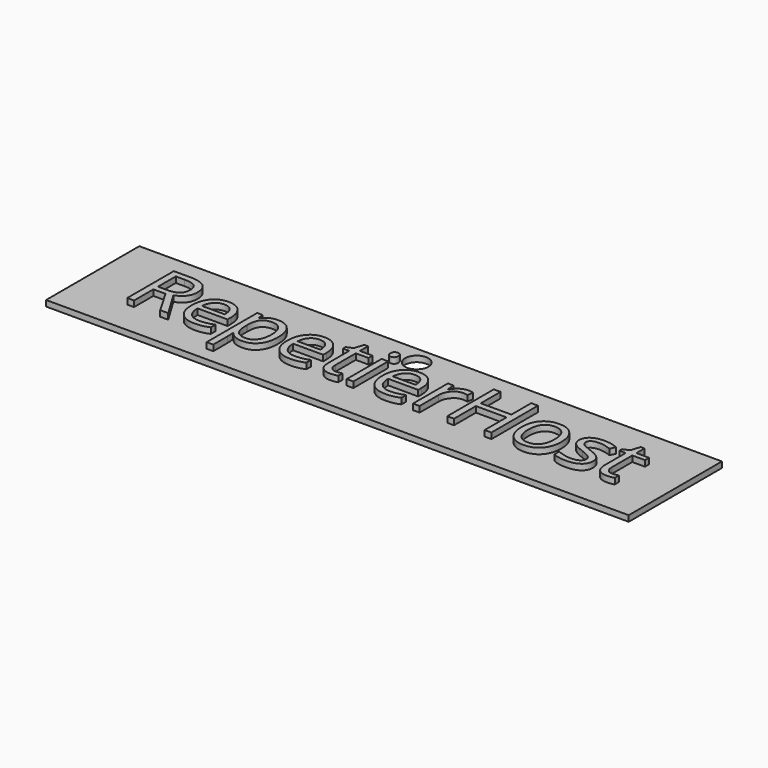
from build123d import *

# Parameters (mm, degrees)
F0_W         = 100
F0_H         = 20
F1_DEPTH     = 1
F2_TEXT_SIZE = 13.9817004215
F3_DEPTH     = 1
F5_D         = 4
F5_DEPTH     = 50
F5_TIP       = 1.2017212381


# Not quite as in the source:
# - Text() gives the source's letters only with a copy of the font that has no kerning and outlines rounded to 1/6400 em; it was checked with that copy


with BuildPart() as f1:
    # F0 (on Top) → F1 (new body)
    with BuildSketch(Plane.XY):
        Rectangle(F0_W, F0_H)
    extrude(amount=F1_DEPTH)

    # F2 (on face) → F3 (join)
    with BuildSketch(Plane.XY.offset(1)):
        with Locations((-42.0372179325, -4.2531144037)):
            Text('RepetierHost', F2_TEXT_SIZE, font='Open Sans', text_align=(TextAlign.LEFT, TextAlign.BOTTOM))
    extrude(amount=F3_DEPTH)

    # F5
    with Locations(Plane.XY.offset(1)):
        with Locations((0.1197934791, 6.8681109697)):
            Hole(F5_D / 2, depth=F5_DEPTH)
            with Locations((0, 0, -(F5_DEPTH + F5_TIP / 2))):  # 118° drill point
                Cone(0, F5_D / 2, F5_TIP, mode=Mode.SUBTRACT)


solid = f1.part
